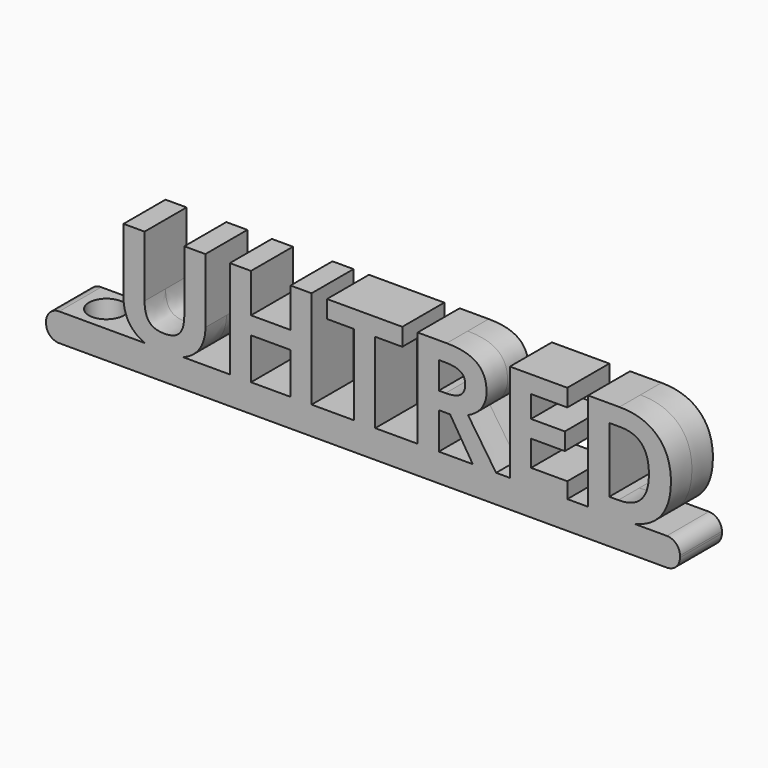
from build123d import *

# Parameters (mm, degrees)
F0_TEXT_SIZE = 15.9809457954
F1_DEPTH     = 3
F2_W         = 65
F2_H         = 6
F3_DEPTH     = 0.2
F4_DEPTH     = 3
F5_W         = 6
F5_H         = 3.2
F6_DEPTH     = 7.5
F7_R         = 1.5
F8_R         = 2
F9_DEPTH     = 3.5
F10_R        = 1.5


# Not quite as in the source:
# - Text() gives the source's letters only with a copy of the font that has no kerning and outlines rounded to 1/6400 em; it was checked with that copy


with BuildPart() as f1:
    # F0 (on Front) → F1 (new body, symmetric)
    with BuildSketch(Plane.XZ):
        with Locations((-20, 0)):
            Text('UHTRED', F0_TEXT_SIZE, font='Open Sans', font_style=FontStyle.BOLD, text_align=(TextAlign.LEFT, TextAlign.BOTTOM))
    extrude(amount=F1_DEPTH, both=True)



with BuildPart() as f3:
    # F2 (on Top) → F3 (new body)
    with BuildSketch(Plane.XY):
        with Locations((12.5, 0)):
            Rectangle(F2_W, F2_H)
    extrude(amount=F3_DEPTH)


with BuildPart() as f4:
    # F4 (new): a face of the model
    f4_faces = [f3.part.faces().sort_by_distance(p)[0] for p in [
        (12.5, 0, 0),
    ]]
    extrude(f4_faces, amount=F4_DEPTH)


with BuildPart() as f1_1:
    add(f1.part)

    add(f3.part)  # F6 merges F3

    add(f4.part)  # F6 merges F4
    # F5 (on face) → F6 (join)
    with BuildSketch(Plane(origin=(-20, 0, 0), x_dir=(0, -1, 0), z_dir=(-1, 0, 0))):
        with Locations((0, -1.4)):
            Rectangle(F5_W, F5_H)
    extrude(amount=F6_DEPTH)

    # F7
    f7_edges = [f1_1.edges().sort_by_distance(p)[0] for p in [
        (-27.5, 0, -3),
        (-27.5, 0, 0.2),
        (45, 0, -3),
    ]]
    fillet(f7_edges, radius=F7_R)

    # F8 (on face) → F9 (cut)
    with BuildSketch(Plane.XY.offset(0.2)):
        with Locations((-23, 0)):
            Circle(F8_R)
    extrude(amount=-F9_DEPTH, mode=Mode.SUBTRACT)

    # F10
    f10_edges = [f1_1.edges().sort_by_distance(p)[0] for p in [
        (45, 0, 0.2),
    ]]
    fillet(f10_edges, radius=F10_R)


solid = f1_1.part
